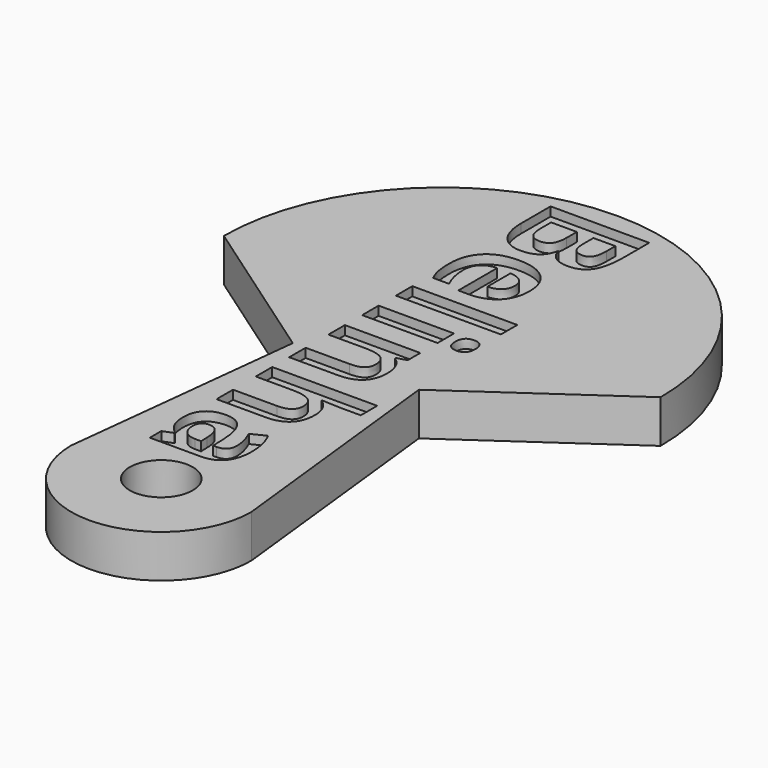
from build123d import *

# Parameters (mm, degrees)
F0_R         = 1.75
F1_DEPTH     = 2.38
F2_TEXT_SIZE = 7.6700553765
F3_DEPTH     = 0.5


# Not quite as in the source:
# - Text() gives the source's letters only with a copy of the font that has no kerning and outlines rounded to 1/6400 em; it was checked with that copy


with BuildPart() as f1:
    # F0 (on Top) → F1 (new body)
    with BuildSketch(Plane.XY):
        with BuildLine():
            Line((3.5, -6), (12.125, 0))
            ThreePointArc((12.125, 0), (0, 12.125), (-12.125, 0))
            Line((-12.125, 0), (-3.5, -6))
            Line((-3.5, -6), (-5, -19.5))
            ThreePointArc((-5, -19.5), (0, -24.5), (5, -19.5))
            Line((5, -19.5), (3.5, -6))
        make_face()
        with Locations((0, -19.5)):
            Circle(F0_R, mode=Mode.SUBTRACT)
    extrude(amount=F1_DEPTH)

    # F2 (on face) → F3 (cut)
    with BuildSketch(Plane.XY.offset(2.38)):
        with Locations(Location((-2.79445636, 11.7), (0, 0, -90))):
            Text('Belinha', F2_TEXT_SIZE, font='Open Sans', font_style=FontStyle.BOLD, text_align=(TextAlign.LEFT, TextAlign.BOTTOM))
    extrude(amount=-F3_DEPTH, mode=Mode.SUBTRACT)


solid = f1.part
